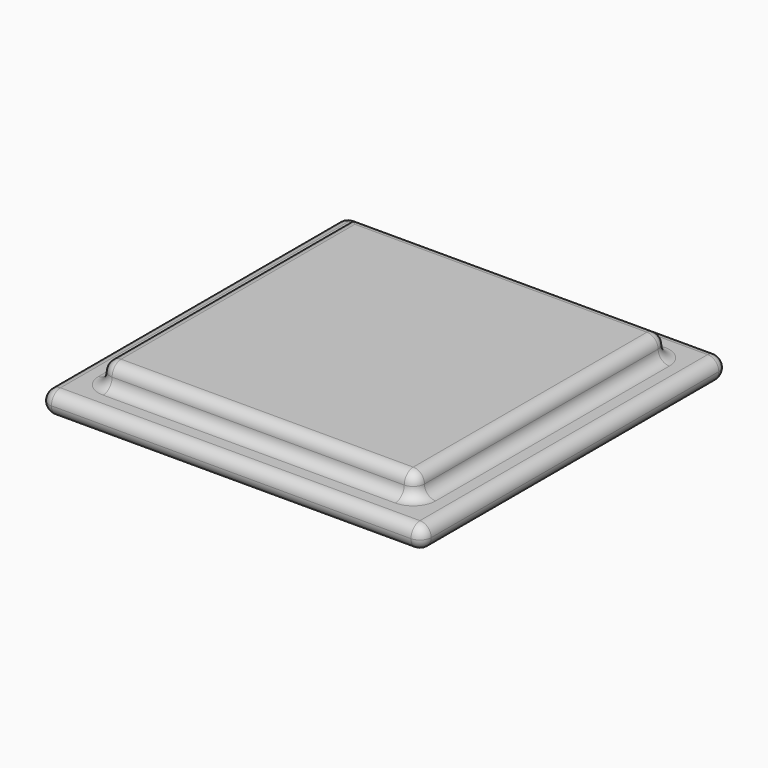
from build123d import *

# Parameters (mm, degrees)
F0_W     = 17
F0_H     = 17
F1_DEPTH = 1
F2_W     = 14
F2_H     = 14
F3_DEPTH = 1
F4_R     = 0.49999


# Not quite as in the source:
# - a fillet or chamfer is up to 0.001 mm smaller than in the source, because OpenCascade refuses the exact size


with BuildPart() as f1:
    # F0 (on Top) → F1 (new body)
    with BuildSketch(Plane.XY):
        with Locations((-37.4565784931, 18.6608627687)):
            Rectangle(F0_W, F0_H)
    extrude(amount=F1_DEPTH)

    # F2 (on face) → F3 (join)
    with BuildSketch(Plane.XY.offset(1)):
        with Locations((-37.4565784931, 18.6608627687)):
            Rectangle(F2_W, F2_H)
    extrude(amount=F3_DEPTH)

    # F4 (radius 0.5 in the source; OpenCascade refuses exactly that, so slightly less here)
    f4_edges = [f1.edges().sort_by_distance(p)[0] for p in [
        (-37.456578, 25.660863, 2),
        (-44.456578, 18.660863, 2),
        (-44.456578, 18.660863, 1),
        (-37.456578, 25.660863, 1),
        (-37.456578, 11.660863, 2),
        (-37.456578, 10.160863, 1),
        (-45.956578, 18.660863, 1),
        (-45.956578, 18.660863, 0),
        (-45.956578, 27.160863, 0.5),
        (-37.456578, 27.160863, 1),
        (-37.456578, 27.160863, 0),
        (-30.456578, 18.660863, 1),
        (-30.456578, 18.660863, 2),
        (-30.456578, 25.660863, 1.5),
        (-28.956578, 18.660863, 1),
        (-28.956578, 18.660863, 0),
        (-28.956578, 27.160863, 0.5),
        (-28.956578, 10.160863, 0.5),
        (-45.956578, 10.160863, 0.5),
        (-37.456578, 10.160863, 0),
        (-37.456578, 11.660863, 1),
        (-44.456578, 11.660863, 1.5),
        (-30.456578, 11.660863, 1.5),
    ]]
    fillet(f4_edges, radius=F4_R)


solid = f1.part
